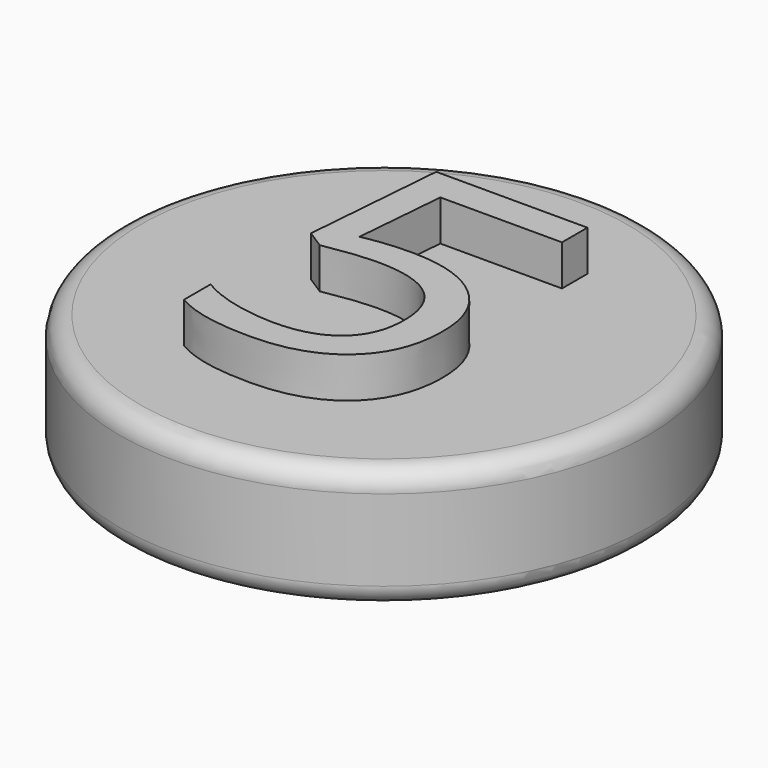
from build123d import *

# Parameters (mm, degrees)
F0_R         = 65
F1_DEPTH     = 30
F2_TEXT_SIZE = 104.8247485111
F3_DEPTH     = 10
F4_R         = 5
F5_R         = 10
F6_DEPTH     = 15


# Not quite as in the source:
# - Text() gives the source's letters only with a copy of the font that has no kerning and outlines rounded to 1/6400 em; it was checked with that copy


with BuildPart() as f1:
    # F0 (on Top) → F1 (new body)
    with BuildSketch(Plane.XY):
        Circle(F0_R)
    extrude(amount=F1_DEPTH)

    # F2 (on face) → F3 (join)
    with BuildSketch(Plane.XY.offset(30)):
        with Locations((-28.7449769676, -37.0919369161)):
            Text('5', F2_TEXT_SIZE, font='Open Sans', text_align=(TextAlign.LEFT, TextAlign.BOTTOM))
    extrude(amount=F3_DEPTH)

    # F4
    f4_edges = [f1.edges().sort_by_distance(p)[0] for p in [
        (-65, 0, 30),
        (65, 0, 15),
        (-65, 0, 0),
    ]]
    fillet(f4_edges, radius=F4_R)

    # F5 (on face) → F6 (join)
    with BuildSketch(Plane(origin=(0, 0, 0), x_dir=(1, 0, 0), z_dir=(0, 0, -1))):
        Circle(F5_R)
    extrude(amount=F6_DEPTH)


solid = f1.part
